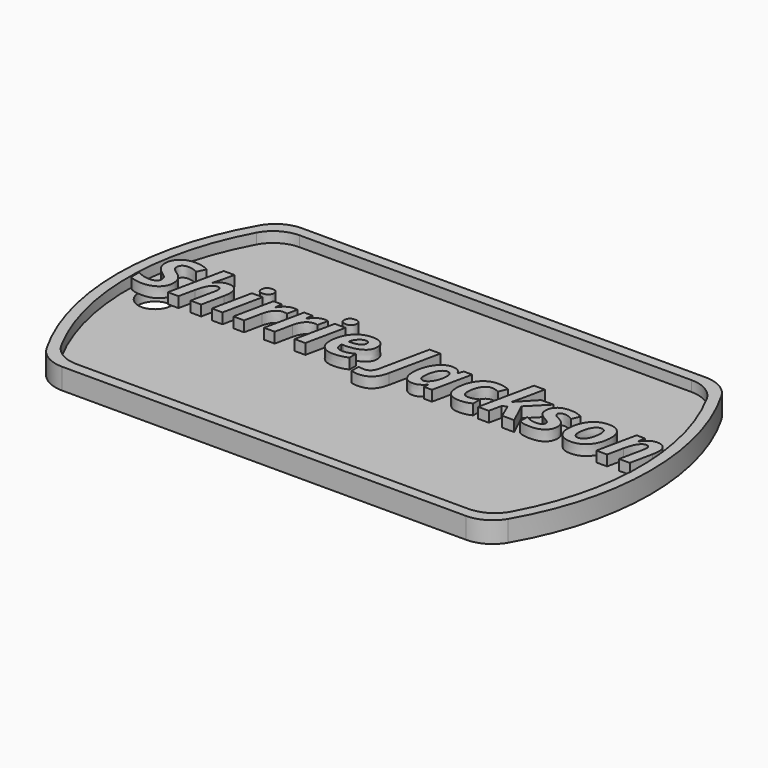
from build123d import *

# Parameters (mm, degrees)
F1_DEPTH     = 1
F3_DEPTH     = 1
F4_R         = 1.5875
F5_DEPTH     = 1
F6_TEXT_SIZE = 6.9328952918
F7_DEPTH     = 1


# Not quite as in the source:
# - Text() gives the source's letters only with a copy of the font that has no kerning and outlines rounded to 1/6400 em; it was checked with that copy


with BuildPart() as f1:
    # F0 (on Top) → F1 (new body)
    with BuildSketch(Plane.XY):
        with BuildLine():
            ThreePointArc((-19.2474145991, 14.2875), (-20.8349145991, 13.862130657), (-21.9970452561, 12.7))
            ThreePointArc((-21.9970452561, 12.7), (-25.4, 0), (-21.9970452561, -12.7))
            ThreePointArc((-21.9970452561, -12.7), (-20.8349145991, -13.862130657), (-19.2474145991, -14.2875))
            Line((-19.2474145991, -14.2875), (19.2474145991, -14.2875))
            ThreePointArc((19.2474145991, -14.2875), (20.8349145991, -13.862130657), (21.9970452561, -12.7))
            ThreePointArc((21.9970452561, -12.7), (25.4, 0), (21.9970452561, 12.7))
            ThreePointArc((21.9970452561, 12.7), (20.8349145991, 13.862130657), (19.2474145991, 14.2875))
            Line((19.2474145991, 14.2875), (-19.2474145991, 14.2875))
        make_face()
    extrude(amount=F1_DEPTH)

    # F2 (on face) → F3 (join)
    with BuildSketch(Plane.XY.offset(1)):
        with BuildLine():
            Line((19.2474145991, 14.2875), (-19.2474145991, 14.2875))
            ThreePointArc((-19.2474145991, 14.2875), (-20.8349145991, 13.862130657), (-21.9970452561, 12.7))
            ThreePointArc((-21.9970452561, 12.7), (-25.4, 0), (-21.9970452561, -12.7))
            ThreePointArc((-21.9970452561, -12.7), (-20.8349145991, -13.862130657), (-19.2474145991, -14.2875))
            Line((-19.2474145991, -14.2875), (19.2474145991, -14.2875))
            ThreePointArc((19.2474145991, -14.2875), (20.8349145991, -13.862130657), (21.9970452561, -12.7))
            ThreePointArc((21.9970452561, -12.7), (25.4, 0), (21.9970452561, 12.7))
            ThreePointArc((21.9970452561, 12.7), (20.8349145991, 13.862130657), (19.2474145991, 14.2875))
        make_face()
        with BuildLine():
            ThreePointArc((-21.4526124879, 11.6252061249), (-20.2856017842, 12.8404540819), (-18.6611352482, 13.2875))
            Line((-18.6611352482, 13.2875), (18.6611352482, 13.2875))
            ThreePointArc((18.6611352482, 13.2875), (20.2856017842, 12.8404540819), (21.4526124879, 11.6252061249))
            ThreePointArc((21.4526124879, 11.6252061249), (24.4, 0), (21.4526124879, -11.6252061249))
            ThreePointArc((21.4526124879, -11.6252061249), (20.2856017842, -12.8404540819), (18.6611352482, -13.2875))
            Line((18.6611352482, -13.2875), (-18.6611352482, -13.2875))
            ThreePointArc((-18.6611352482, -13.2875), (-20.2856017842, -12.8404540819), (-21.4526124879, -11.6252061249))
            ThreePointArc((-21.4526124879, -11.6252061249), (-24.4, 0), (-21.4526124879, 11.6252061249))
        make_face(mode=Mode.SUBTRACT)
    extrude(amount=F3_DEPTH)

    # F4 (on face) → F5 (cut)
    with BuildSketch(Plane.XY.offset(1)):
        with Locations((-21.821282804, 0)):
            Circle(F4_R)
    extrude(amount=-F5_DEPTH, mode=Mode.SUBTRACT)

    # F6 (on face) → F7 (join)
    with BuildSketch(Plane.XY.offset(1)):
        with Locations((-24.4, 0)):
            Text('Shirrie Jackson', F6_TEXT_SIZE, font='Open Sans', font_style=FontStyle.BOLDITALIC, text_align=(TextAlign.LEFT, TextAlign.BOTTOM))
    extrude(amount=F7_DEPTH)


solid = f1.part
